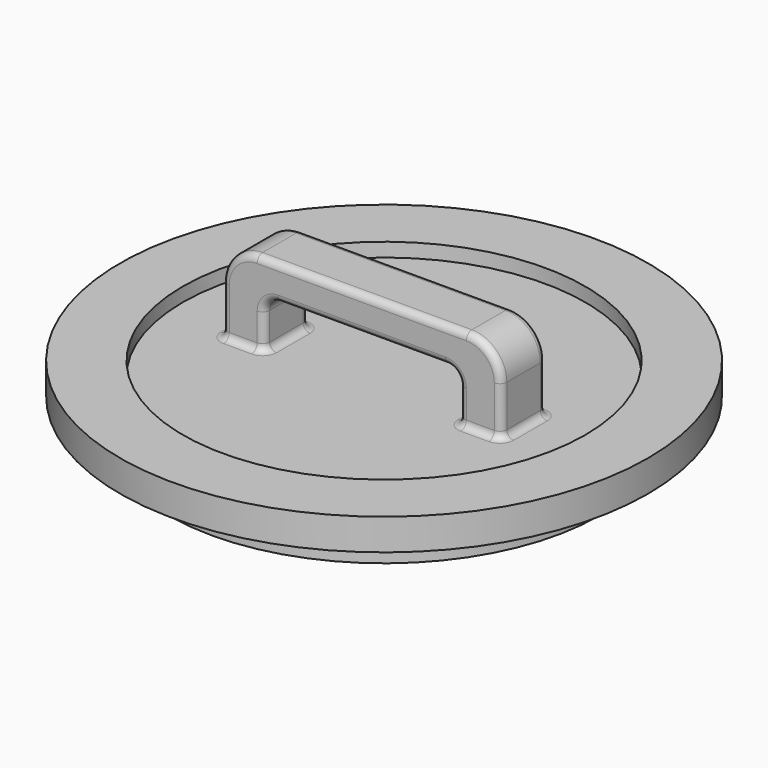
from build123d import *

# Parameters (mm, degrees)
F1_R      = 30.9
F2_DEPTH  = 5
F3_R      = 37.85
F4_DEPTH  = 4.5
F5_R      = 28.85
F6_DEPTH  = 2
F7_W      = 40
F7_H      = 8
F9_DEPTH  = 12
F10_R     = 5
F8_W      = 28
F8_H      = 8
F11_DEPTH = 7
F12_R     = 2
F13_F1_R  = 1
F13_F2_R  = 1


with BuildPart() as f2:
    # F1 (on offset) → F2 (new body)
    with BuildSketch(Plane.XY):
        Circle(F1_R)
    extrude(amount=F2_DEPTH)

    # F3 (on face) → F4 (join)
    with BuildSketch(Plane.XY.offset(5)):
        Circle(F3_R)
    extrude(amount=F4_DEPTH)

    # F5 (on face) → F6 (cut)
    with BuildSketch(Plane.XY.offset(9.5)):
        Circle(F5_R)
    extrude(amount=-F6_DEPTH, mode=Mode.SUBTRACT)

    # F7 (on face) → F9 (join)
    with BuildSketch(Plane.XY.offset(7.5)):
        Rectangle(F7_W, F7_H)
    extrude(amount=F9_DEPTH)

    # F10
    f10_edges = [f2.edges().sort_by_distance(p)[0] for p in [
        (-20, 0, 19.5),
        (20, 0, 19.5),
    ]]
    fillet(f10_edges, radius=F10_R)

    # F8 (on face) → F11 (cut)
    with BuildSketch(Plane.XY.offset(7.5)):
        Rectangle(F8_W, F8_H)
    extrude(amount=F11_DEPTH, mode=Mode.SUBTRACT)

    # F12
    f12_edges = [f2.edges().sort_by_distance(p)[0] for p in [
        (-14, 0, 14.5),
        (14, 0, 14.5),
    ]]
    fillet(f12_edges, radius=F12_R)

    # F13: fillet of radius 1 on 24 edges, made by hand

    # F13_f1
    f13_f1_edges = [f2.edges().sort_by_distance(p)[0] for p in [
        (0, -4, 19.5),
        (14, -4, 10),
        (13.4142135624, -4, 13.9142135624),
        (0, -4, 14.5),
        (-13.4142135624, -4, 13.9142135624),
        (-14, -4, 10),
        (-20, -4, 11),
        (-18.5355339059, -4, 18.0355339059),
        (18.5355339059, -4, 18.0355339059),
        (20, -4, 11),
        (14, 4, 10),
        (13.4142135624, 4, 13.9142135624),
        (0, 4, 14.5),
        (20, 4, 11),
        (-13.4142135624, 4, 13.9142135624),
        (18.5355339059, 4, 18.0355339059),
        (-14, 4, 10),
        (0, 4, 19.5),
        (-18.5355339059, 4, 18.0355339059),
        (-20, 4, 11),
    ]]
    fillet(f13_f1_edges, radius=F13_F1_R)

    # F13_f2
    f13_f2_edges = [f2.edges().sort_by_distance(p)[0] for p in [
        (-17, -4, 7.5),
        (17, -4, 7.5),
        (17, 4, 7.5),
        (-17, 4, 7.5),
        (-14.2928932188, 3.7071067812, 7.5),
        (-19.7071067812, 3.7071067812, 7.5),
        (19.7071067812, 3.7071067812, 7.5),
        (14.2928932188, 3.7071067812, 7.5),
        (14.2928932188, -3.7071067812, 7.5),
        (19.7071067812, -3.7071067812, 7.5),
        (-19.7071067812, -3.7071067812, 7.5),
        (-14.2928932188, -3.7071067812, 7.5),
    ]]
    fillet(f13_f2_edges, radius=F13_F2_R)


solid = f2.part
